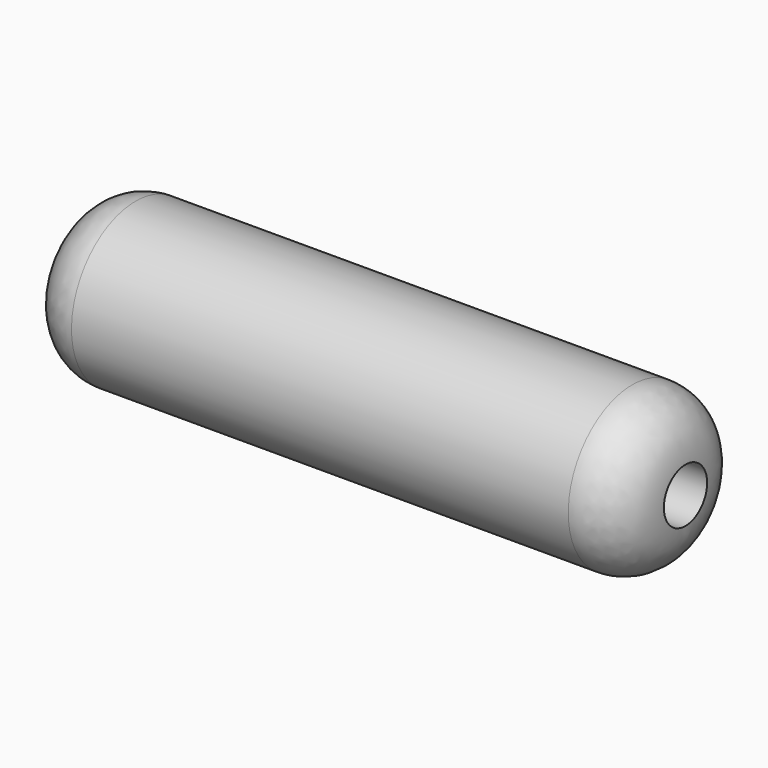
from build123d import *


# Not quite as in the source:
# - a fillet or chamfer that OpenCascade refuses, or shapes differently, is made with other operations: its cross-section is extruded or revolved along the edge and cut away or added


with BuildPart() as f2:
    # F0 (on Front) → F2 (revolve)
    with BuildSketch(Plane.XZ):
        Polygon((2.5167669653, 0), (0, 0), (0, -9.5830742138), (72.0989203059, -9.5830742138), (72.0989203059, -3.2330742138), (2.5167669653, -3.2330742138), align=None)
    revolve(axis=Axis((32.417844981, 0, 0), (1, 0, 0)))

    # F3: fillet of radius 6.35 on 2 edges, made by hand

    # F3_s1 → F3_t2 (revolve, cut)
    with BuildSketch(Plane.XZ):
        with BuildLine():
            ThreePointArc((0, -3.2330742138), (1.8598719395, -7.7232022744), (6.35, -9.5830742138))
            Line((6.35, -9.5830742138), (0, -9.5830742138))
            Line((0, -9.5830742138), (0, -3.2330742138))
        make_face()
    revolve(axis=Axis((0, 0, 0), (1, 0, 0)), mode=Mode.SUBTRACT)

    # F3_s3 → F3_t4 (revolve, cut)
    with BuildSketch(Plane.XZ):
        with BuildLine():
            ThreePointArc((65.7489203059, -9.5830742138), (70.2390483664, -7.7232022744), (72.0989203059, -3.2330742138))
            Line((72.0989203059, -3.2330742138), (72.0989203059, -9.5830742138))
            Line((72.0989203059, -9.5830742138), (65.7489203059, -9.5830742138))
        make_face()
    revolve(axis=Axis((72.0989203059, 0, 0), (1, 0, 0)), mode=Mode.SUBTRACT)


solid = f2.part
